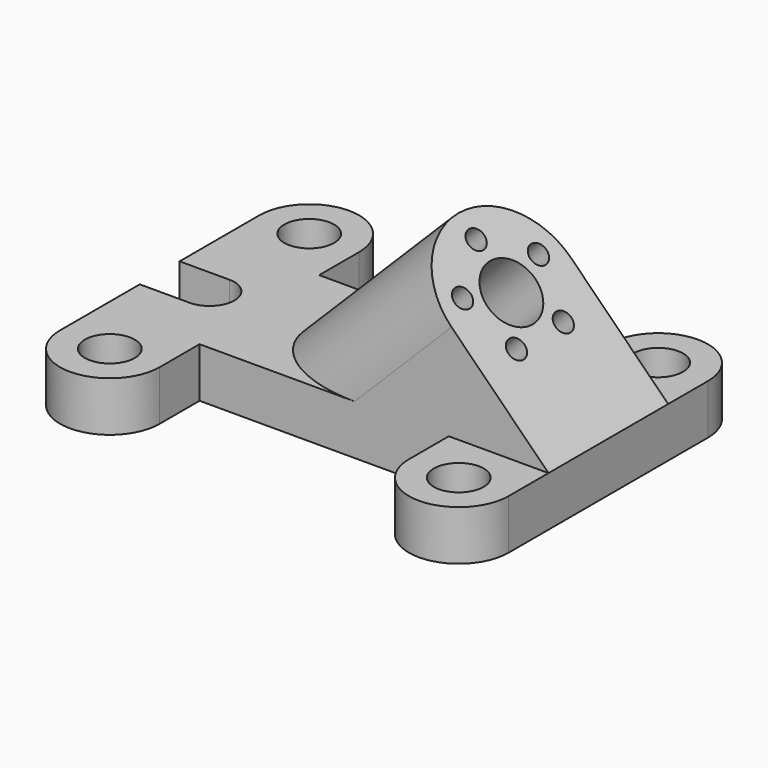
from build123d import *

# Parameters (mm, degrees)
F1_DEPTH          = 12.7
F2_R              = 6.35
F3_DEPTH          = 12.701
F8_R              = 7.62
F9_DEPTH          = 89.8035612107
F10_R             = 2.54
F11_DEPTH         = 6.35
F11_COPIES_COUNT  = 2
F11_COPIES_PITCH  = 14.929745
F11_COPIES1_COUNT = 2
F11_COPIES1_PITCH = 14.929745
F11_COPIES2_COUNT = 2
F11_COPIES2_PITCH = 24.156836
F11_COPIES3_COUNT = 2
F11_COPIES3_PITCH = 24.156836


# Not quite as in the source:
# - a pattern or mirror of a feature is missing from the dataset's text; its kind, count and spacing are read off the source's solid


with BuildPart() as f1:
    # F0 (on Top) → F1 (new body)
    with BuildSketch(Plane.XY):
        with BuildLine():
            Line((63.5, 0), (0, 0))
            Line((0, 0), (0, 12.7))
            ThreePointArc((0, 12.7), (-12.7, 25.4), (-25.4, 12.7))
            Line((-25.4, 12.7), (-25.4, -12.7))
            Line((-25.4, -12.7), (-12.7, -12.7))
            ThreePointArc((-12.7, -12.7), (-6.35, -19.05), (-12.7, -25.4))
            Line((-12.7, -25.4), (-25.4, -25.4))
            Line((-25.4, -25.4), (-25.4, -50.8))
            ThreePointArc((-25.4, -50.8), (-12.7, -63.5), (0, -50.8))
            Line((0, -50.8), (0, -38.1))
            Line((0, -38.1), (63.5, -38.1))
            Line((63.5, -38.1), (63.5, -50.8))
            ThreePointArc((63.5, -50.8), (76.2, -63.5), (88.9, -50.8))
            Line((88.9, -50.8), (88.9, 12.7))
            ThreePointArc((88.9, 12.7), (76.2, 25.4), (63.5, 12.7))
            Line((63.5, 12.7), (63.5, 0))
        make_face()
    extrude(amount=F1_DEPTH)

    # F2 (on face) → F3 (cut, through all)
    with BuildSketch(Plane.XY.offset(12.7)):
        with Locations((-12.7, 12.7)):
            Circle(F2_R)
        with Locations((76.2, 12.7)):
            Circle(F2_R)
        with Locations((76.2, -50.8)):
            Circle(F2_R)
        with Locations((-12.7, -50.8)):
            Circle(F2_R)
    extrude(amount=-F3_DEPTH, mode=Mode.SUBTRACT)

    # F6 (on face) → F7 (join, up to the next surface of F1)
    with BuildSketch(Plane(origin=(50.8, 0, 50.8), x_dir=(0, 1, 0), z_dir=(0.7071067812, 0, 0.7071067812))):
        with BuildLine():
            Line((-38.1, -18.9565367084), (-38.1, -53.8815367264))
            Line((-38.1, -53.8815367264), (0, -53.8815367264))
            Line((0, -53.8815367264), (0, -18.9565360082))
            ThreePointArc((0, -18.9565360082), (-19.0500003501, 0.0934632736), (-38.1, -18.9565367084))
        make_face()
    extrude(until=Until.NEXT, dir=(-0.7071067812, 0, -0.7071067812))

    # F8 (on face) → F9 (cut, through all)
    with BuildSketch(Plane(origin=(50.8, 0, 50.8), x_dir=(0, 1, 0), z_dir=(0.7071067812, 0, 0.7071067812))):
        with Locations((-19.05, -18.9565367264)):
            Circle(F8_R)
    extrude(amount=-F9_DEPTH, mode=Mode.SUBTRACT)

    # F10 (on face) → F11 (cut)
    with BuildSketch(Plane(origin=(50.8, 0, 50.8), x_dir=(0, 1, 0), z_dir=(0.7071067812, 0, 0.7071067812))):
        with Locations((-19.05, -6.2565367264)):
            Circle(F10_R)
    f11 = extrude(amount=-F11_DEPTH, mode=Mode.SUBTRACT)

    # F11_copies: F11 ×2
    with Locations(*[Vector(0.4156269378, -0.8090169944, -0.4156269378) * (i * F11_COPIES_PITCH) for i in range(1, F11_COPIES_COUNT)]):
        add(f11, mode=Mode.SUBTRACT)

    # F11_copies1: F11 ×2
    with Locations(*[Vector(0.4156269378, 0.8090169944, -0.4156269378) * (i * F11_COPIES1_PITCH) for i in range(1, F11_COPIES1_COUNT)]):
        add(f11, mode=Mode.SUBTRACT)

    # F11_copies2: F11 ×2
    with Locations(*[Vector(0.672498512, 0.3090169944, -0.672498512) * (i * F11_COPIES2_PITCH) for i in range(1, F11_COPIES2_COUNT)]):
        add(f11, mode=Mode.SUBTRACT)

    # F11_copies3: F11 ×2
    with Locations(*[Vector(0.672498512, -0.3090169944, -0.672498512) * (i * F11_COPIES3_PITCH) for i in range(1, F11_COPIES3_COUNT)]):
        add(f11, mode=Mode.SUBTRACT)


solid = f1.part
